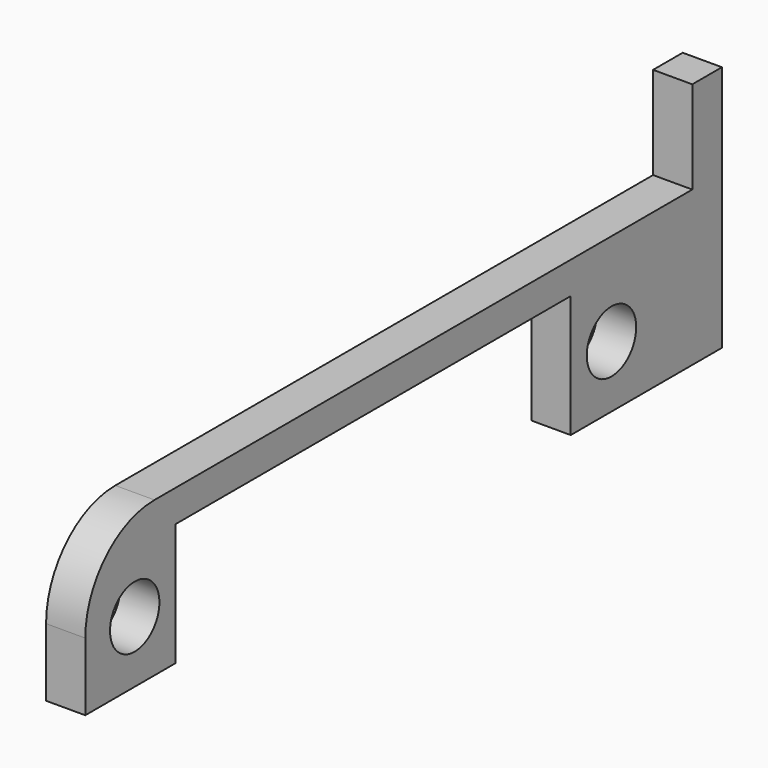
from build123d import *

# Parameters (mm, degrees)
F0_R     = 2.5
F1_DEPTH = 3.175
F2_R     = 7


# Not quite as in the source:
# - a length typed as a fraction of an inch, garbled in the dataset ("3 / 203.2 mm" for 3/8 in), is restored


with BuildPart() as f1:
    # F0 (on Right) → F1 (new body)
    with BuildSketch(Plane.YZ):
        Polygon((-9.125, 0), (0, 0), (0, 9.91), (20, 9.91), (40, 9.91), (40, 0), (52.3, 0), (55.3, 0), (55.3, 20), (52.3, 20), (52.3, 12.5), (-9.125, 12.5), align=None)
        with Locations((-4.125, 5)):
            Circle(F0_R, mode=Mode.SUBTRACT)
        with Locations((44.125, 5)):
            Circle(F0_R, mode=Mode.SUBTRACT)
    extrude(amount=F1_DEPTH)

    # F2
    f2_edges = [f1.edges().sort_by_distance(p)[0] for p in [
        (1.5875, -9.125, 12.5),
    ]]
    fillet(f2_edges, radius=F2_R)


solid = f1.part
